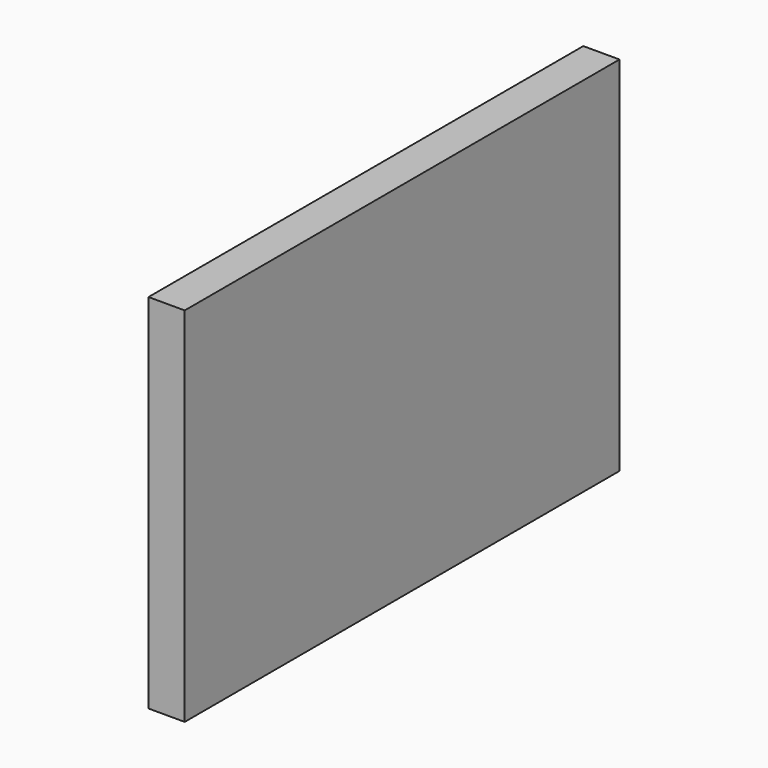
from build123d import *

# Parameters (mm, degrees)
F0_W     = 76.2
F0_H     = 50.79353787
F3_DEPTH = 5.08


# Not quite as in the source:
# - the program builds the solid bodies; features that only make, move or delete a surface that nothing else refers to are left out


with BuildPart() as f3:
    # F0 (on Right) → F3 (new body)
    with BuildSketch(Plane.YZ):
        with Locations((2.5172638655, 9.6503077075)):
            Rectangle(F0_W, F0_H)
    extrude(amount=-F3_DEPTH)


solid = f3.part
